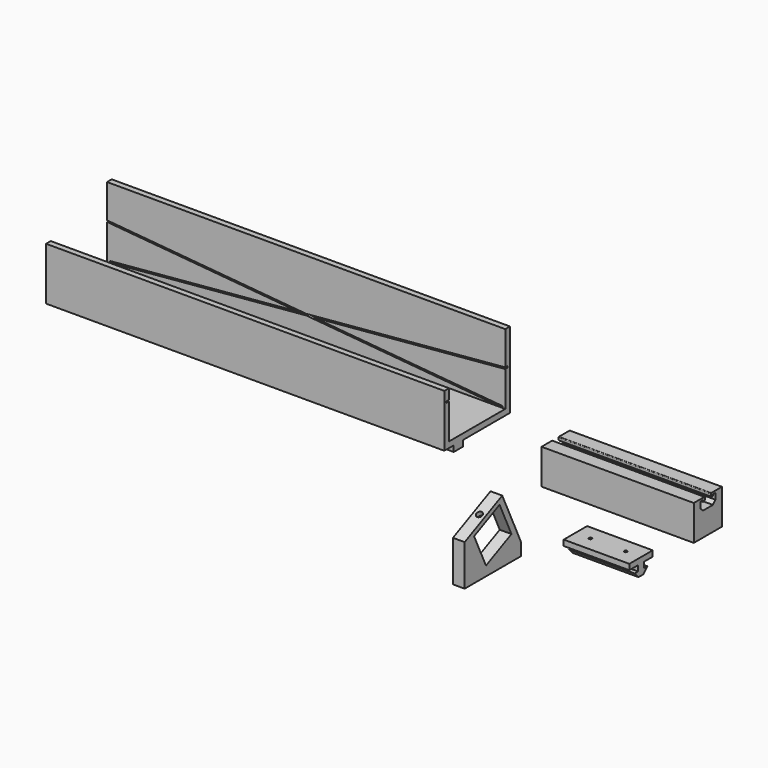
from build123d import *

# Parameters (mm, degrees)
F0_W          = 38.1
F0_H          = 38.1
F1_DEPTH      = 165.1
F2_W          = 431.8
F2_H          = 6.35
F2_H_2        = 76.2
F3_DEPTH      = 6.35
F4_W          = 431.8
F4_H          = 6.35
F5_DEPTH      = 76.2
F6_W          = 431.8
F6_H          = 6.35
F7_DEPTH      = 50.8
F9_DEPTH      = 3.175
F9_DEPTH_BACK = 79.375
F10_W         = 431.8
F10_H         = 12.7
F11_DEPTH     = 6.35
F13_DEPTH     = 12.7
F14_DEPTH     = 44.45
F16_DEPTH     = 12.7
F17_R         = 3.175
F18_DEPTH     = 5.08
F20_DEPTH     = 165.1
F21_R         = 0.79375
F23_DEPTH     = 71.12
F24_R         = 1.5875
F25_DEPTH     = 17.78
F26_R         = 1.5875
F27_DEPTH     = 6.35
F29_DEPTH     = 12.7


# Not quite as in the source:
# - a feature names something its author has since deleted; it is built from what else it names


with BuildPart() as f1:
    # F0 (on Right) → F1 (new body)
    with BuildSketch(Plane.YZ):
        with Locations((19.05, 19.05)):
            Rectangle(F0_W, F0_H)
    extrude(amount=F1_DEPTH)

    # F19 (on face) → F20 (cut, through all)
    with BuildSketch(Plane.YZ.offset(165.1)):
        with BuildLine():
            Line((12.4706910076, 25.7937), (19.05, 25.7937))
            Line((19.05, 25.7937), (25.6293089924, 25.7937))
            ThreePointArc((25.6293089924, 25.7937), (25.7811864797, 25.8239103105), (25.9099419962, 25.9099419962))
            Line((25.9099419962, 25.9099419962), (29.2207580038, 29.2207580038))
            ThreePointArc((29.2207580038, 29.2207580038), (29.3067896895, 29.3495135203), (29.337, 29.5013910076))
            Line((29.337, 29.5013910076), (29.337, 35.493325))
            ThreePointArc((29.337, 35.493325), (29.2207580038, 35.7739580038), (28.940125, 35.8902))
            Line((28.940125, 35.8902), (26.190575, 35.8902))
            ThreePointArc((26.190575, 35.8902), (25.9099419962, 35.7739580038), (25.7937, 35.493325))
            Line((25.7937, 35.493325), (25.7937, 34.432875))
            ThreePointArc((25.7937, 34.432875), (25.6774580038, 34.1522419962), (25.396825, 34.036))
            Line((25.396825, 34.036), (24.7015, 34.036))
            ThreePointArc((24.7015, 34.036), (23.5789679849, 34.5009679849), (23.114, 35.6235))
            Line((23.114, 35.6235), (23.114, 38.1))
            Line((23.114, 38.1), (19.05, 38.1))
            Line((19.05, 38.1), (14.986, 38.1))
            Line((14.986, 38.1), (14.986, 35.6235))
            ThreePointArc((14.986, 35.6235), (14.5210320151, 34.5009679849), (13.3985, 34.036))
            Line((13.3985, 34.036), (12.703175, 34.036))
            ThreePointArc((12.703175, 34.036), (12.4225419962, 34.1522419962), (12.3063, 34.432875))
            Line((12.3063, 34.432875), (12.3063, 35.493325))
            ThreePointArc((12.3063, 35.493325), (12.1900580038, 35.7739580038), (11.909425, 35.8902))
            Line((11.909425, 35.8902), (9.159875, 35.8902))
            ThreePointArc((9.159875, 35.8902), (8.8792419962, 35.7739580038), (8.763, 35.493325))
            Line((8.763, 35.493325), (8.763, 29.5013910076))
            ThreePointArc((8.763, 29.5013910076), (8.7932103105, 29.3495135203), (8.8792419962, 29.2207580038))
            Line((8.8792419962, 29.2207580038), (12.1900580038, 25.9099419962))
            ThreePointArc((12.1900580038, 25.9099419962), (12.3188135203, 25.8239103105), (12.4706910076, 25.7937))
        make_face()
    extrude(amount=-F20_DEPTH, mode=Mode.SUBTRACT)

    # F21
    f21_edges = [f1.edges().sort_by_distance(p)[0] for p in [
        (82.55, 14.986, 38.1),
        (82.55, 23.114, 38.1),
    ]]
    fillet(f21_edges, radius=F21_R)


with BuildPart() as f3:
    # F2 (on Top) → F3 (new body)
    with BuildSketch(Plane.XY):
        with Locations((-321.2767546883, 3.175)):
            Rectangle(F2_W, F2_H)
        with Locations((-321.2767546883, 44.45)):
            Rectangle(F2_W, F2_H_2)
        with Locations((-321.2767546883, 85.725)):
            Rectangle(F2_W, F2_H)
    extrude(amount=F3_DEPTH)

    # F4 (on face) → F5 (join)
    with BuildSketch(Plane.XY.offset(6.35)):
        with Locations((-321.2767546883, 85.725)):
            Rectangle(F4_W, F4_H)
    extrude(amount=F5_DEPTH)

    # F6 (on face) → F7 (join)
    with BuildSketch(Plane.XY.offset(6.35)):
        with Locations((-321.2767546883, 3.175)):
            Rectangle(F6_W, F6_H)
    extrude(amount=F7_DEPTH)

    # F8 (on face) → F9 (cut, two sides)
    with BuildSketch(Plane.XZ.offset(-82.55)) as f9_sk:
        Polygon((-537.1767546883, 44.45), (-330.3075385094, 26.1968338666), (-321.2767546883, 26.9936677331), (-537.1767546883, 46.0436677331), align=None)
        Polygon((-321.2767546883, 26.9936677331), (-312.2459708672, 26.1968338666), (-105.3767546883, 44.45), (-105.3767546883, 46.0436677331), align=None)
        Polygon((-321.2767546883, 25.4), (-108.678998386, 6.6413744439), (-108.5394669621, 8.2227305808), (-312.2459708672, 26.1968338666), align=None)
        Polygon((-330.3075385094, 26.1968338666), (-321.2767546883, 25.4), (-312.2459708672, 26.1968338666), (-321.2767546883, 26.9936677331), align=None)
        Polygon((-533.8745109906, 6.6413744439), (-321.2767546883, 25.4), (-330.3075385094, 26.1968338666), (-534.0140424144, 8.2227305808), align=None)
    extrude(amount=-F9_DEPTH, mode=Mode.SUBTRACT)
    extrude(f9_sk.sketch, amount=F9_DEPTH_BACK, mode=Mode.SUBTRACT)

    # F10 (on face) → F11 (join)
    with BuildSketch(Plane(origin=(0, 0, 0), x_dir=(1, 0, 0), z_dir=(0, 0, -1))):
        with Locations((-321.2767546883, -19.05)):
            Rectangle(F10_W, F10_H)
    extrude(amount=F11_DEPTH)

    # F26 (on face) → F27 (cut, through all)
    with BuildSketch(Plane.XY.offset(6.35)):
        with Locations((-302.2267546883, 57.15)):
            Circle(F26_R)
        with Locations((-340.3267546883, 57.15)):
            Circle(F26_R)
    extrude(amount=-F27_DEPTH, mode=Mode.SUBTRACT)


with BuildPart() as f13:
    # F12 (on Right) → F13 (new body)
    with BuildSketch(Plane.YZ):
        Polygon((-120.0692180491, 0), (-43.8692180491, 0), (-43.8692180491, 35.5326435514), align=None)
    extrude(amount=F13_DEPTH)

    # F14 (add): a face of the model
    f14_faces = [f13.faces().sort_by_distance(p)[0] for p in [
        (6.35, -81.9692180491, 0),
    ]]
    extrude(f14_faces, amount=F14_DEPTH)

    # F15 (on face) → F16 (cut, through all)
    with BuildSketch(Plane.YZ.offset(12.7)):
        Polygon((-56.6531768199, -18.0724728657), (-72.7549325922, 16.4578538203), (-107.2852592783, 0.356098048), (-91.1835035059, -34.1742286381), align=None)
    extrude(amount=-F16_DEPTH, mode=Mode.SUBTRACT)

    # F17 (on face) → F18 (cut, through all)
    with BuildSketch(Plane(origin=(0, -19.2982054215, 41.3851350799), x_dir=(1, 0, 0), z_dir=(0, 0.4226182617, -0.906307787))):
        with Locations((6.35, 78.0329723801)):
            Circle(F17_R)
    extrude(amount=-F18_DEPTH, mode=Mode.SUBTRACT)

    # F28 (on face) → F29 (cut, through all)
    with BuildSketch(Plane.YZ.offset(12.7)):
        Polygon((-43.8692180491, 35.5326435514), (-69.1467789141, 23.7455233405), (-43.8692180491, -30.4623808682), align=None)
    extrude(amount=-F29_DEPTH, mode=Mode.SUBTRACT)


with BuildPart() as f23:
    # F22 (on Right) → F23 (new body)
    with BuildSketch(Plane.YZ):
        Polygon((61.7622073192, -62.7286910119), (30.0122073192, -62.7286910119), (30.0122073192, -68.8246910119), (42.0772073192, -68.8246910119), (42.0772073192, -74.9206910119), (37.3147073192, -74.9206910119), (42.4582073192, -80.5086910119), (49.3162073192, -80.5086910119), (54.4597073192, -74.9206910119), (49.6972073192, -74.9206910119), (49.6972073192, -68.8246910119), (61.7622073192, -68.8246910119), align=None)
    extrude(amount=F23_DEPTH)

    # F24 (on face) → F25 (cut, through all)
    with BuildSketch(Plane(origin=(0, 0, -80.5086910119), x_dir=(1, 0, 0), z_dir=(0, 0, -1))):
        with Locations((54.4576, -45.8872073192)):
            Circle(F24_R)
        with Locations((16.3576, -45.8872073192)):
            Circle(F24_R)
    extrude(amount=-F25_DEPTH, mode=Mode.SUBTRACT)


solid = Compound([f1.part, f3.part, f13.part, f23.part])
